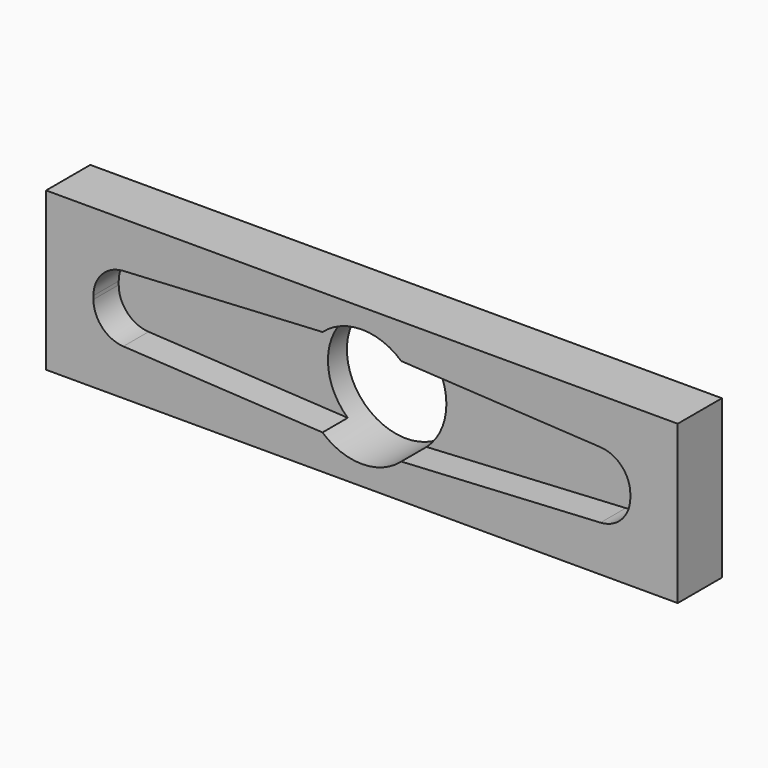
from build123d import *

# Parameters (mm, degrees)
F0_W     = 40
F0_H     = 10
F0_R     = 3.75
F1_DEPTH = 3.5
F3_DEPTH = 2


# Not quite as in the source:
# - a pattern or mirror of a feature is missing from the dataset's text; its kind, count and spacing are read off the source's solid


with BuildPart() as f1:
    # F0 (on Front) → F1 (new body)
    with BuildSketch(Plane.XZ):
        with Locations((20, 7.299159328)):
            Rectangle(F0_W, F0_H)
        with Locations((20, 7.299159328)):
            Circle(F0_R, mode=Mode.SUBTRACT)
    extrude(amount=F1_DEPTH)

    # F2 (on face) → F3 (cut)
    with BuildSketch(Plane.XZ.offset(3.5)):
        with BuildLine():
            ThreePointArc((17.5055060633, 4.499159328), (16.25, 7.299159328), (17.5055060633, 10.099159328))
            Line((17.5055060633, 10.099159328), (4.8898644293, 9.4033881317))
            ThreePointArc((4.8898644293, 9.4033881317), (3.5473694307, 8.7811462961), (3, 7.4064228951))
            Line((3, 7.4064228951), (3, 7.1918957609))
            ThreePointArc((3, 7.1918957609), (3.5473694307, 5.8171723599), (4.8898644293, 5.1949305243))
            Line((4.8898644293, 5.1949305243), (17.5055060633, 4.499159328))
        make_face()
    f3 = extrude(amount=-F3_DEPTH, mode=Mode.SUBTRACT)

    # F3_copies: F3 across plane
    add(f3.mirror(Plane(origin=(20, 0, 0), x_dir=(0, 0, 1), z_dir=(1, 0, 0))), mode=Mode.SUBTRACT)


solid = f1.part
